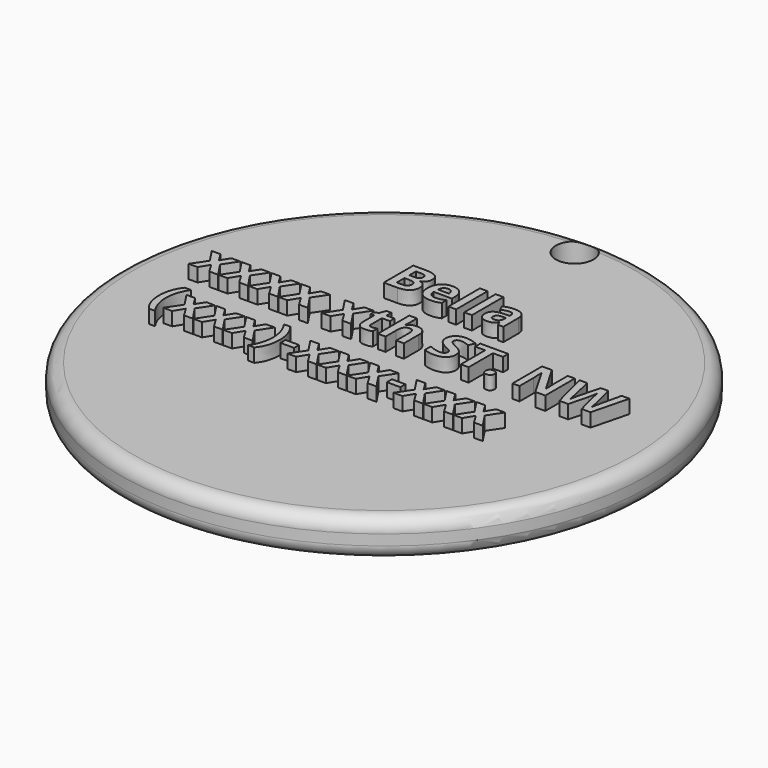
from build123d import *

# Parameters (mm, degrees)
F0_R         = 44.45
F1_DEPTH     = 3.175
F2_R         = 3.175
F3_DEPTH     = 12.7
F6_TEXT_SIZE = 8.7082886919
F7_DEPTH     = 2.286


# Not quite as in the source:
# - a fillet or chamfer that OpenCascade refuses, or shapes differently, is made with other operations: its cross-section is extruded or revolved along the edge and cut away or added
# - Text() gives the source's letters only with a copy of the font that has no kerning and outlines rounded to 1/6400 em; it was checked with that copy


with BuildPart() as f1:
    # F0 (on Top) → F1 (new body, symmetric)
    with BuildSketch(Plane.XY):
        Circle(F0_R)
    extrude(amount=F1_DEPTH, both=True)

    # F2 (on Top) → F3 (cut, symmetric)
    with BuildSketch(Plane.XY):
        with Locations((0, 40.1277458341)):
            Circle(F2_R)
    extrude(amount=F3_DEPTH, both=True, mode=Mode.SUBTRACT)

    # F5: fillet of radius 2.286 on 2 edges, made by hand

    # F5_s1 → F5_t2 (revolve, cut)
    with BuildSketch(Plane.XZ):
        with BuildLine():
            ThreePointArc((44.45, 0.889), (43.7804461018, 2.5054461018), (42.164, 3.175))
            Line((42.164, 3.175), (44.45, 3.175))
            Line((44.45, 3.175), (44.45, 0.889))
        make_face()
    revolve(axis=Axis((0, 0, 3.175), (0, 0, 1)), mode=Mode.SUBTRACT)

    # F5_s3 → F5_t4 (revolve, cut)
    with BuildSketch(Plane.XZ):
        with BuildLine():
            ThreePointArc((44.45, -0.889), (43.7804461018, -2.5054461018), (42.164, -3.175))
            Line((42.164, -3.175), (44.45, -3.175))
            Line((44.45, -3.175), (44.45, -0.889))
        make_face()
    revolve(axis=Axis((0, 0, -3.175), (0, 0, 1)), mode=Mode.SUBTRACT)

    # F6 (on face) → F7 (join)
    with BuildSketch(Plane.XY.offset(3.175)):
        with Locations((-12.2970561021, 14.3242327551)):
            Text('Bella', F6_TEXT_SIZE, font='Open Sans', font_style=FontStyle.BOLD, text_align=(TextAlign.LEFT, TextAlign.BOTTOM))
        with Locations((-34.925, 2.4809601341)):
            Text('xxxx xth ST. NW', F6_TEXT_SIZE, font='Open Sans', font_style=FontStyle.BOLD, text_align=(TextAlign.LEFT, TextAlign.BOTTOM))
        with Locations((-32.6622056102, -9.362312487)):
            Text('(xxx)-xxx-xxx', F6_TEXT_SIZE, font='Open Sans', font_style=FontStyle.BOLD, text_align=(TextAlign.LEFT, TextAlign.BOTTOM))
    extrude(amount=F7_DEPTH)


solid = f1.part
